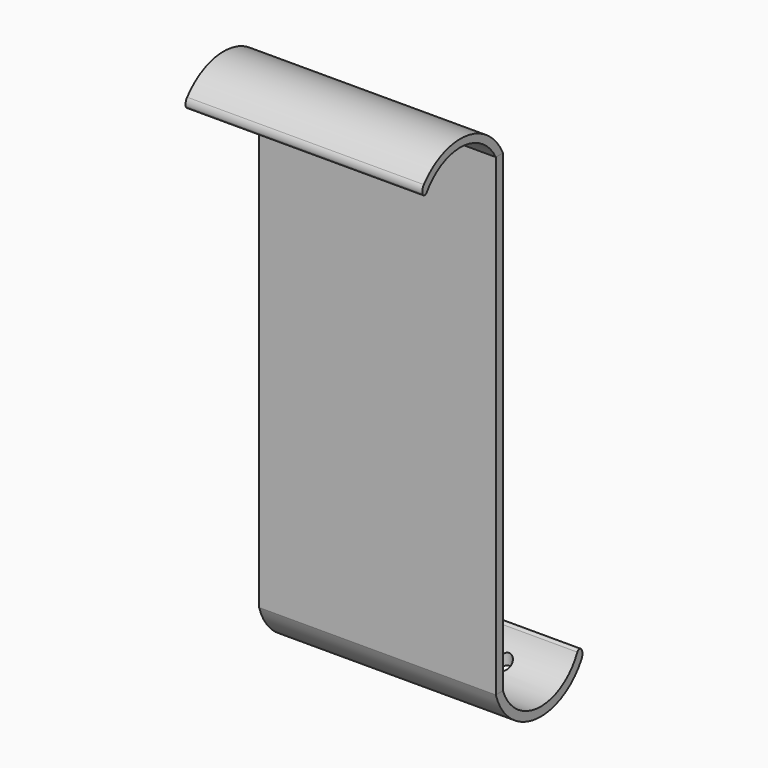
from build123d import *

# Parameters (mm, degrees)
F0_W          = 80
F0_H          = 160
F1_DEPTH      = 3
F3_DEPTH      = 80
F4_T1_DEPTH   = 104.5932134922
F4_2_T1_DEPTH = 102.506788887
F5_R          = 1
F5_2_R        = 1
F6_R          = 2.5
F7_DEPTH      = 139.3101269636


# Not quite as in the source:
# - a fillet or chamfer that OpenCascade refuses, or shapes differently, is made with other operations: its cross-section is extruded or revolved along the edge and cut away or added


with BuildPart() as f1:
    # F0 (on Front) → F1 (new body)
    with BuildSketch(Plane.XZ):
        with Locations((-7.3579295626, -45.1037270249)):
            Rectangle(F0_W, F0_H)
    extrude(amount=F1_DEPTH)


with BuildPart() as f3:
    # F2 (on face) → F3 (new body)
    with BuildSketch(Plane.YZ.offset(32.6420704374)):
        with BuildLine():
            Line((-3, 34.8962729751), (0, 34.8962729751))
            ThreePointArc((0, 34.8962729751), (-17.9972580969, 46.4620537988), (-35.9945161939, 34.8962729751))
            Line((-35.9945161939, 34.8962729751), (-32.9945161939, 34.8962729751))
            ThreePointArc((-32.9945161939, 34.8962729751), (-17.9972580969, 43.8911340273), (-3, 34.8962729751))
        make_face()
    extrude(amount=-F3_DEPTH)

    # F4: fillet of radius 3 on 1 edges, made by hand

    # F4_s2 → F4_t1 (cut)
    with BuildSketch(Plane.YZ.offset(-59.6545363087)):
        with BuildLine():
            ThreePointArc((-33.4108326759, 39.0816792247), (-34.0589945612, 36.9037991395), (-32.9945161939, 34.8962729751))
            Line((-32.9945161939, 34.8962729751), (-35.9945161939, 34.8962729751))
            ThreePointArc((-35.9945161939, 34.8962729751), (-34.8332416261, 37.0695762328), (-33.4108326759, 39.0816792247))
        make_face()
    extrude(amount=F4_T1_DEPTH, mode=Mode.SUBTRACT)

    # F5
    f5_edges = [f3.edges().sort_by_distance(p)[0] for p in [
        (-7.35793, -32.994516, 34.896273),
    ]]
    fillet(f5_edges, radius=F5_R)


with BuildPart() as f3b:
    # F2 (on face) → F3, piece 2 (new body)
    with BuildSketch(Plane.YZ.offset(32.6420704374)):
        with BuildLine():
            ThreePointArc((31.9638926898, -125.1037270249), (15.9819463449, -136.3091268636), (0, -125.1037270249))
            Line((0, -125.1037270249), (-3, -125.1037270249))
            ThreePointArc((-3, -125.1037270249), (15.9819463449, -139.3091268636), (34.9638926898, -125.1037270249))
            Line((34.9638926898, -125.1037270249), (31.9638926898, -125.1037270249))
        make_face()
    extrude(amount=-F3_DEPTH)

    # F4#2: fillet of radius 3 on 1 edges, made by hand

    # F4_2_s2 → F4_2_t1 (cut)
    with BuildSketch(Plane.YZ.offset(-58.6113240061)):
        with BuildLine():
            ThreePointArc((33.2114216404, -129.2499381943), (33.4716947989, -126.9108397557), (31.9638926898, -125.1037270249))
            Line((31.9638926898, -125.1037270249), (34.9638926898, -125.1037270249))
            ThreePointArc((34.9638926898, -125.1037270249), (34.2059560867, -127.2268337858), (33.2114216404, -129.2499381943))
        make_face()
    extrude(amount=F4_2_T1_DEPTH, mode=Mode.SUBTRACT)

    # F5#2
    f5_2_edges = [f3b.edges().sort_by_distance(p)[0] for p in [
        (-7.35793, 31.963893, -125.103727),
    ]]
    fillet(f5_2_edges, radius=F5_2_R)

    # F6 (on Top) → F7 (cut, through all)
    with BuildSketch(Plane.XY):
        with Locations((12.6420704374, 25.2114216404)):
            Circle(F6_R)
    extrude(amount=-F7_DEPTH, mode=Mode.SUBTRACT)


solid = Compound([f1.part, f3.part, f3b.part])
